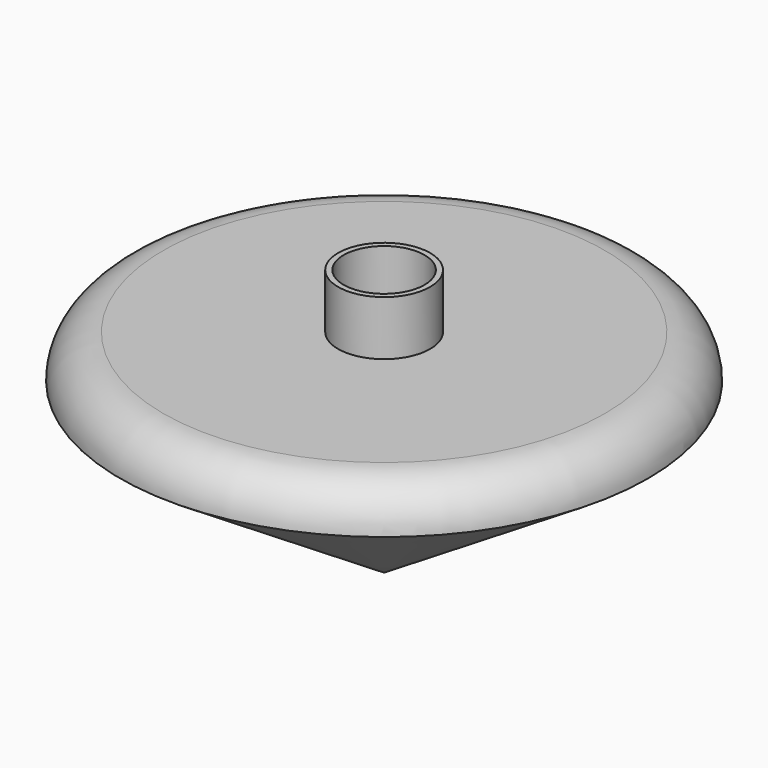
from build123d import *

# Parameters (mm, degrees)
F2_R     = 4.7625
F3_DEPTH = 9.525
F4_R     = 5.07999


# Not quite as in the source:
# - a fillet or chamfer is up to 0.001 mm smaller than in the source, because OpenCascade refuses the exact size


with BuildPart() as f1:
    # F0 (on Front) → F1 (revolve)
    with BuildSketch(Plane.XZ):
        Polygon((0, 31.392690606), (0, 0), (31.0912281275, 19.8785602432), (31.0912281275, 24.9585602432), (5.4195728153, 24.9585602432), (5.4195728153, 31.392690606), align=None)
    revolve(axis=Axis((0, 0, 15.696345303), (0, 0, -1)))

    # F2 (on face) → F3 (cut)
    with BuildSketch(Plane.XY.offset(31.392690606)):
        Circle(F2_R)
    extrude(amount=-F3_DEPTH, mode=Mode.SUBTRACT)

    # F4 (radius 5.08 in the source; OpenCascade refuses exactly that, so slightly less here)
    f4_edges = [f1.edges().sort_by_distance(p)[0] for p in [
        (-31.091228, 0, 24.95856),
    ]]
    fillet(f4_edges, radius=F4_R)


solid = f1.part
